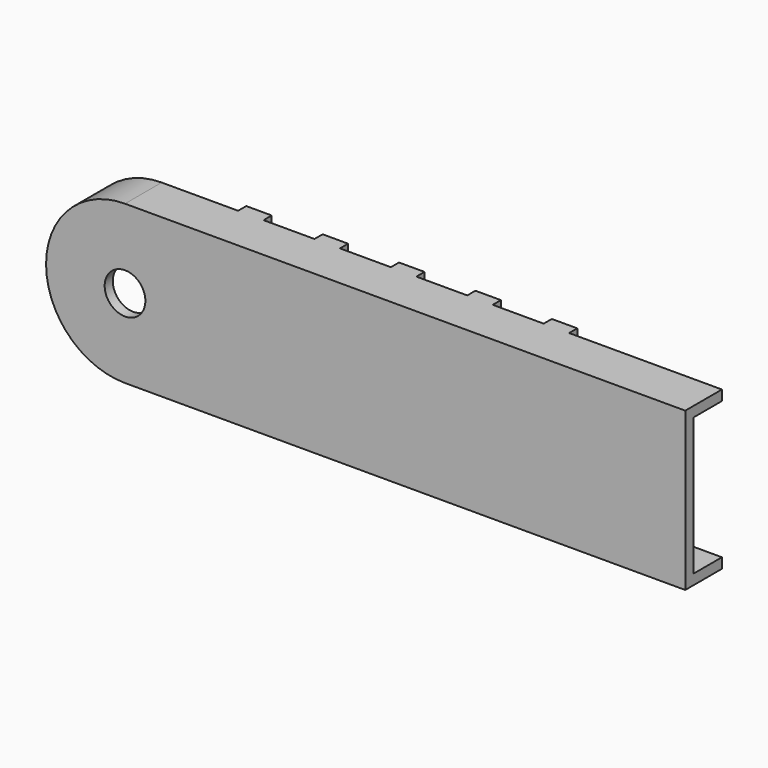
from build123d import *

# Parameters (mm, degrees)
F1_DEPTH = 7
F2_T     = 2
F3_D     = 8
F4_W     = 5
F4_H     = 2
F5_DEPTH = 2


# Not quite as in the source:
# - a feature of the source that left no trace in its solid (it failed there, or was rolled back) is left out


with BuildPart() as f1:
    # F0 (on Front) → F1 (new body)
    with BuildSketch(Plane.XZ):
        with BuildLine():
            ThreePointArc((0, -13.5), (9.545941546, -9.545941546), (13.5, 0))
            ThreePointArc((13.5, 0), (9.545941546, 9.545941546), (0, 13.5))
            Line((0, 13.5), (0, -13.5))
        make_face()
        with BuildLine():
            ThreePointArc((0, 13.5), (9.545941546, 9.545941546), (13.5, 0))
            ThreePointArc((13.5, 0), (9.545941546, -9.545941546), (0, -13.5))
            Line((0, -13.5), (110, -13.5))
            Line((110, -13.5), (110, 13.5))
            Line((110, 13.5), (0, 13.5))
        make_face()
        with BuildLine():
            Line((0, -13.5), (0, 13.5))
            ThreePointArc((0, 13.5), (-13.5, 0), (0, -13.5))
        make_face()
    extrude(amount=F1_DEPTH)

    # F2
    f2_openings = [f1.faces().sort_by_distance(p)[0] for p in [
        (49.660922, 0, 0),
        (110, -3.5, 0),
    ]]
    offset(amount=F2_T, openings=f2_openings, kind=Kind.INTERSECTION)

    # F3 (through all)
    with Locations(Plane(origin=(0, 0, 0), x_dir=(1, 0, 0), z_dir=(0, 1, 0))):
        with Locations((0, 0)):
            Hole(F3_D / 2)

    # F4 (on face) → F5 (join)
    with BuildSketch(Plane(origin=(0, 0, 0), x_dir=(-1, 0, 0), z_dir=(0, 1, 0))):
        with Locations((-17.5, -14.5)):
            Rectangle(F4_W, F4_H)
        with BuildLine():
            Line((-20, -13.5), (-15, -13.5))
            ThreePointArc((-15, -13.5), (-17.5, -11), (-20, -13.5))
        make_face()
        with Locations((-32.5, -14.5)):
            Rectangle(F4_W, F4_H)
        with BuildLine():
            Line((-35, -13.5), (-30, -13.5))
            ThreePointArc((-30, -13.5), (-32.5, -11), (-35, -13.5))
        make_face()
        with Locations((-47.5, -14.5)):
            Rectangle(F4_W, F4_H)
        with BuildLine():
            Line((-50, -13.5), (-45, -13.5))
            ThreePointArc((-45, -13.5), (-47.5, -11), (-50, -13.5))
        make_face()
        with Locations((-62.5, -14.5)):
            Rectangle(F4_W, F4_H)
        with BuildLine():
            Line((-65, -13.5), (-60, -13.5))
            ThreePointArc((-60, -13.5), (-62.5, -11), (-65, -13.5))
        make_face()
        with Locations((-77.5, -14.5)):
            Rectangle(F4_W, F4_H)
        with BuildLine():
            Line((-80, -13.5), (-75, -13.5))
            ThreePointArc((-75, -13.5), (-77.5, -11), (-80, -13.5))
        make_face()
        with Locations((-17.5, 14.5)):
            Rectangle(F4_W, F4_H)
        with BuildLine():
            ThreePointArc((-20, 13.5), (-17.5, 11), (-15, 13.5))
            Line((-15, 13.5), (-20, 13.5))
        make_face()
        with BuildLine():
            ThreePointArc((-35, 13.5), (-32.5, 11), (-30, 13.5))
            Line((-30, 13.5), (-35, 13.5))
        make_face()
        with Locations((-32.5, 14.5)):
            Rectangle(F4_W, F4_H)
        with BuildLine():
            ThreePointArc((-50, 13.5), (-47.5, 11), (-45, 13.5))
            Line((-45, 13.5), (-50, 13.5))
        make_face()
        with Locations((-47.5, 14.5)):
            Rectangle(F4_W, F4_H)
        with BuildLine():
            ThreePointArc((-65, 13.5), (-62.5, 11), (-60, 13.5))
            Line((-60, 13.5), (-65, 13.5))
        make_face()
        with Locations((-62.5, 14.5)):
            Rectangle(F4_W, F4_H)
        with BuildLine():
            ThreePointArc((-80, 13.5), (-77.5, 11), (-75, 13.5))
            Line((-75, 13.5), (-80, 13.5))
        make_face()
        with Locations((-77.5, 14.5)):
            Rectangle(F4_W, F4_H)
    extrude(amount=F5_DEPTH)


solid = f1.part
